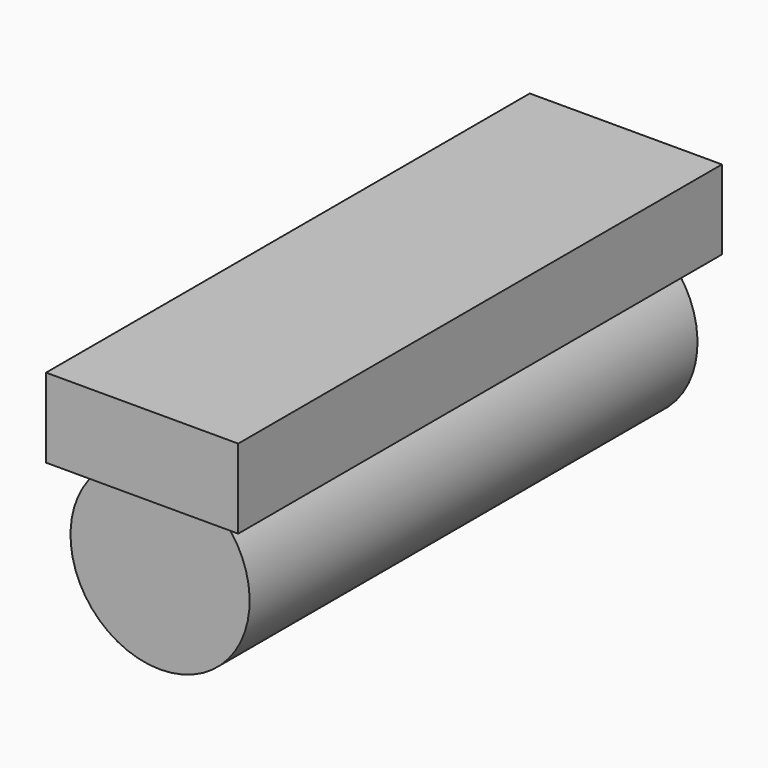
from build123d import *

# Parameters (mm, degrees)
F1_DEPTH = 25
F3_DEPTH = 25
F5_DEPTH = 25
F7_DEPTH = 3.5409905045


with BuildPart() as f1:
    # F0 (on Front) → F1 (new body)
    with BuildSketch(Plane.XZ):
        with BuildLine():
            Line((2.4765, 3.141169806), (-2.4765, 3.141169806))
            ThreePointArc((-2.4765, 3.141169806), (0, -4), (2.4765, 3.141169806))
        make_face()
    extrude(amount=-F1_DEPTH)


with BuildPart() as f3:
    # F2 (on face) → F3 (new body)
    with BuildSketch(Plane.XZ):
        with BuildLine():
            ThreePointArc((-1, 3.8729833462), (-1.7763447939, 3.583936268), (-2.4765, 3.141169806))
            Line((-2.4765, 3.141169806), (2.4765, 3.141169806))
            ThreePointArc((2.4765, 3.141169806), (1.7763447939, 3.583936268), (1, 3.8729833462))
            Line((1, 3.8729833462), (1, 5.141169806))
            Line((1, 5.141169806), (-1, 5.141169806))
            Line((-1, 5.141169806), (-1, 3.8729833462))
        make_face()
    extrude(amount=-F3_DEPTH)


with BuildPart() as f5:
    # F4 (on face) → F5 (new body)
    with BuildSketch(Plane.XZ):
        with BuildLine():
            Line((-1, 3.8729833462), (-1, 5.141169806))
            Line((-1, 5.141169806), (1, 5.141169806))
            Line((1, 5.141169806), (1, 3.8729833462))
            ThreePointArc((1, 3.8729833462), (1.7763447939, 3.583936268), (2.4765, 3.141169806))
            Line((2.4765, 3.141169806), (4.2906352319, 3.141169806))
            Line((4.2906352319, 3.141169806), (4.2906352319, 6.6821603104))
            Line((4.2906352319, 6.6821603104), (0, 6.6821603104))
            Line((0, 6.6821603104), (-4.2906352319, 6.6821603104))
            Line((-4.2906352319, 6.6821603104), (-4.2906352319, 3.141169806))
            Line((-4.2906352319, 3.141169806), (-2.4765, 3.141169806))
            ThreePointArc((-2.4765, 3.141169806), (-1.7763447939, 3.583936268), (-1, 3.8729833462))
        make_face()
    extrude(amount=-F5_DEPTH)

    # F6 (on face) → F7 (join, through all)
    with BuildSketch(Plane(origin=(0, 0, 3.141169806), x_dir=(1, 0, 0), z_dir=(0, 0, -1))):
        Polygon((-4.2906352319, 0), (-2.4765, 0), (2.4765, 0), (4.2906352319, 0), (4.2906352319, 1), (-4.2906352319, 1), align=None)
        Polygon((2.4765, -25), (-2.4765, -25), (-4.2906352319, -25), (-4.2906352319, -26), (4.2906352319, -26), (4.2906352319, -25), align=None)
    extrude(amount=-F7_DEPTH)


solid = Compound([f1.part, f3.part, f5.part])
